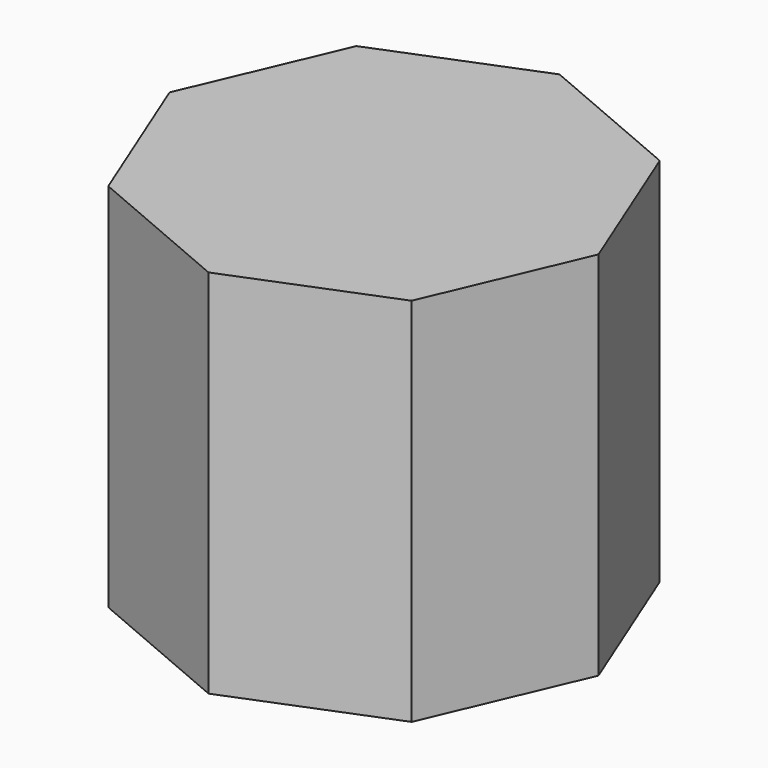
from build123d import *

# Parameters (mm, degrees)
F3_DEPTH = 39.116


# Not quite as in the source:
# - the program builds the solid bodies; features that only make, move or delete a surface that nothing else refers to are left out


with BuildPart() as f3:
    # F2 (on Top) → F3 (new body)
    with BuildSketch(Plane.XY):
        Polygon((22.8255171269, -0.2510304161), (16.317583254, 15.962572635), (0.2510304161, 22.8255171269), (-15.962572635, 16.317583254), (-22.8255171269, 0.2510304161), (-16.317583254, -15.962572635), (-0.2510304161, -22.8255171269), (15.962572635, -16.317583254), align=None)
    extrude(amount=F3_DEPTH)


solid = f3.part
